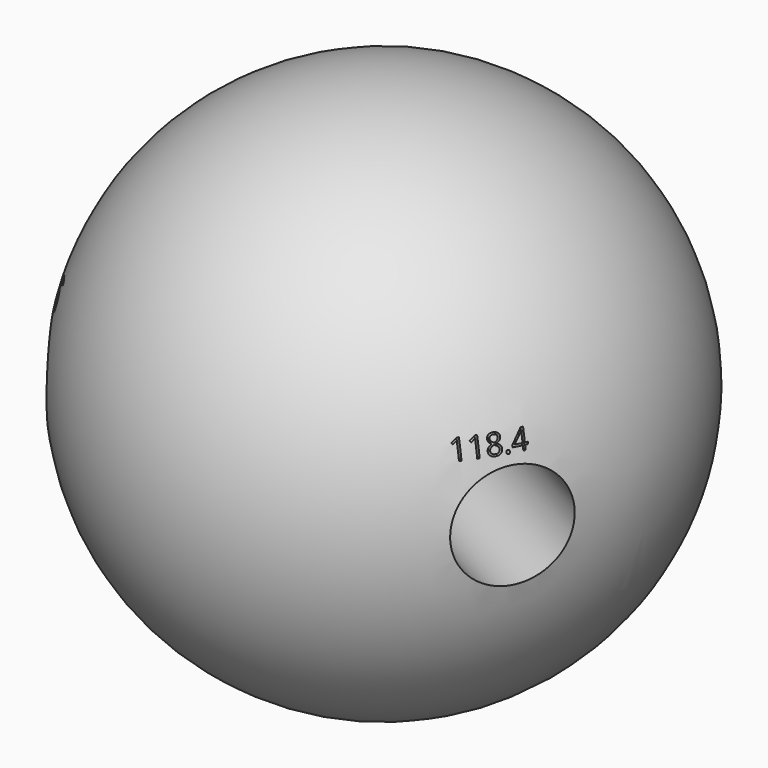
from build123d import *

# Parameters (mm, degrees)
F4_R          = 3.175
F5_DEPTH      = 25.4
F7_TEXT_SIZE  = 1.4580967319
F8_DEPTH      = 10.16
F10_ANGLE     = 118.4
F12_TEXT_SIZE = 1.5362903165
F13_DEPTH     = 10.16
F15_ANGLE     = -122.5
F17_TEXT_SIZE = 2.3977446189
F18_DEPTH     = 10.16


# Not quite as in the source:
# - Text() gives the source's letters only with a copy of the font that has no kerning and outlines rounded to 1/6400 em; it was checked with that copy


with BuildPart() as f2:
    # F0 (on Front) → F2 (revolve)
    with BuildSketch(Plane.XZ):
        with BuildLine():
            Line((15.875, 0), (-15.875, 0))
            ThreePointArc((-15.875, 0), (0, -15.875), (15.875, 0))
        make_face()
    revolve(axis=Axis((0, 0, 0), (1, 0, 0)))

    # F7 (on offset) → F8 (cut)
    with BuildSketch(Plane(origin=(0, 19.05, 0), x_dir=(-1, 0, 0), z_dir=(0, 1, 0))):
        with Locations((-1.8484671891, 3.6443956196)):
            Text('119.1', F7_TEXT_SIZE, font='Open Sans', text_align=(TextAlign.LEFT, TextAlign.BOTTOM))
    extrude(amount=-F8_DEPTH, mode=Mode.SUBTRACT)

    # F12 (on offset) → F13 (cut)
    with BuildSketch(Plane(origin=(16.7573053131, -9.0606411828, 0), x_dir=(0.4756242091, 0.8796485729, 0), z_dir=(0.8796485729, -0.4756242091, 0))):
        with Locations((-2.9949415475, 3.7389001809)):
            Text('118.4', F12_TEXT_SIZE, font='Open Sans', text_align=(TextAlign.LEFT, TextAlign.BOTTOM))
    extrude(amount=-F13_DEPTH, mode=Mode.SUBTRACT)

    # F17 (on offset) → F18 (cut)
    with BuildSketch(Plane(origin=(-16.0666070427, -10.235557539, 0), x_dir=(0.5372996083, -0.8433914458, 0), z_dir=(-0.8433914458, -0.5372996083, 0))):
        with Locations((-4.5452793129, 3.4652657341)):
            Text('122.5', F17_TEXT_SIZE, font='Open Sans', text_align=(TextAlign.LEFT, TextAlign.BOTTOM))
    extrude(amount=-F18_DEPTH, mode=Mode.SUBTRACT)


with BuildPart() as f5:
    # F4 (on offset) → F5 (new body)
    with BuildSketch(Plane.XZ.offset(-6.35)):
        Circle(F4_R)
    extrude(amount=-F5_DEPTH)


with BuildPart() as f10_1:
    # F10: copy of F5
    add(f5.part.rotate(Axis((0, 0, -5.807178095), (0, 0, -1)), F10_ANGLE))


with BuildPart() as f15_1:
    # F15: copy of F5
    add(f5.part.rotate(Axis((0, 0, -0.8295979351), (0, 0, -1)), F15_ANGLE))


with BuildPart() as f2_1:
    add(f2.part)

    # F19: cut F5, F15_1, F10_1
    add(f5.part, mode=Mode.SUBTRACT)
    add(f15_1.part, mode=Mode.SUBTRACT)
    add(f10_1.part, mode=Mode.SUBTRACT)


solid = f2_1.part
